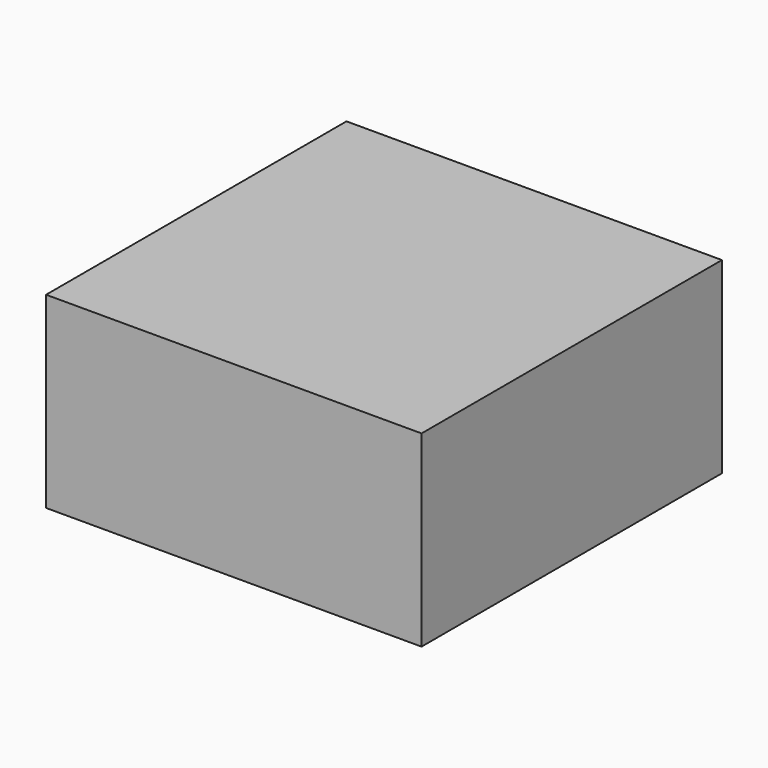
from build123d import *

# Parameters (mm, degrees)
F3_W     = 20
F3_H     = 20
F4_DEPTH = 10
F5_W     = 19.58
F5_H     = 19.58
F6_DEPTH = 9.1


# Not quite as in the source:
# - a feature names something its author has since deleted; it is built from what else it names


with BuildPart() as f4:
    # F3 (on Top) → F4 (new body)
    with BuildSketch(Plane.XY):
        Rectangle(F3_W, F3_H)
    extrude(amount=F4_DEPTH)

    # F5 (on face) → F6 (cut, through all)
    with BuildSketch(Plane(origin=(0, 0, 0), x_dir=(1, 0, 0), z_dir=(0, 0, -1))):
        with Locations((-0.21, -0.21)):
            Rectangle(F5_W, F5_H)
    extrude(amount=-F6_DEPTH, mode=Mode.SUBTRACT)


solid = f4.part
